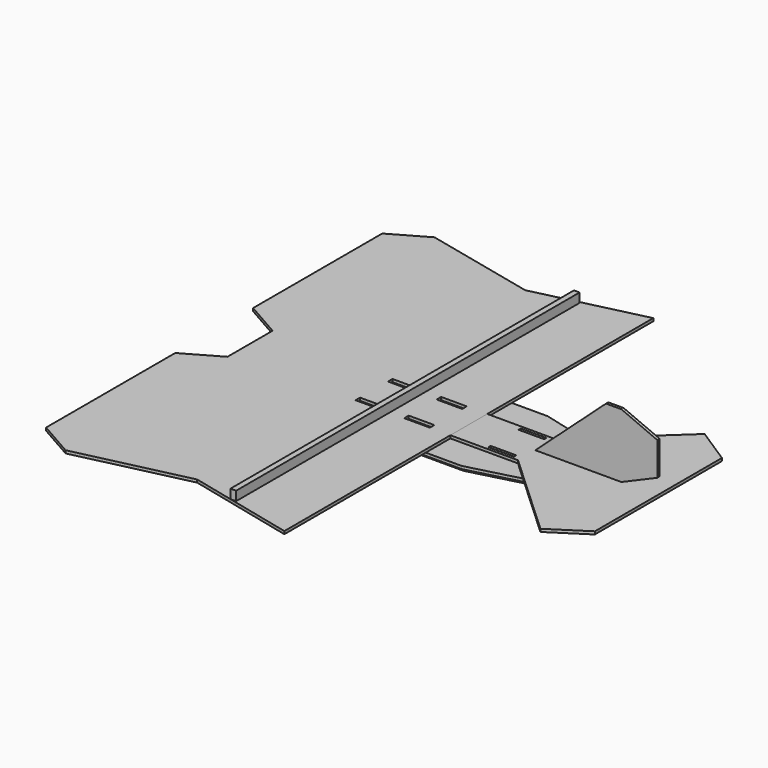
from build123d import *

# Parameters (mm, degrees)
F0_W      = 11
F0_H      = 50
F0_W_2    = 50
F0_H_2    = 11
F1_DEPTH  = 5.5
F2_W      = 11
F2_H      = 94.0476190476
F2_H_2    = 50
F2_H_3    = 110
F2_H_4    = 230
F3_DEPTH  = 18
F4_DEPTH  = 5.5
F5_W      = 50
F5_H      = 5.5
F5_W_2    = 120
F5_H_2    = 60
F6_DEPTH  = 5.5
F8_DEPTH  = 5.5
F9_W      = 50
F9_H      = 5.5
F9_W_2    = 40
F10_DEPTH = 5.5
F11_W     = 40
F11_H     = 5.5
F11_W_2   = 48
F11_W_3   = 20
F12_DEPTH = 125
F13_DEPTH = 5.5
F15_DEPTH = 5.5
F16_W     = 50
F16_H     = 5.5
F17_DEPTH = 5.5


# Not quite as in the source:
# - a feature names something its author has since deleted; it is built from what else it names


with BuildPart() as f1:
    # F0 (on Top) → F1 (new body)
    with BuildSketch(Plane.XY):
        Polygon((0, -400), (0, 0), (0, 400), (-217, 450), (-217, 400), (-217, 55), (-217, -55), (-217, -450), align=None)
        Polygon((-217, 400), (-217, 450), (-287, 410), (-287, 95), (-217, 55), align=None)
        Polygon((0, 400), (0, 0), (0, -400), (210, -450), (210, 0), (210, 450), align=None)
        with Locations((85.5, -300)):
            Rectangle(F0_W, F0_H, mode=Mode.SUBTRACT)
        with Locations((85.5, -140)):
            Rectangle(F0_W, F0_H, mode=Mode.SUBTRACT)
        with Locations((50, -39.5)):
            Rectangle(F0_W_2, F0_H_2, mode=Mode.SUBTRACT)
        with Locations((145, -39.5)):
            Rectangle(F0_W_2, F0_H_2, mode=Mode.SUBTRACT)
        with Locations((50, 39.5)):
            Rectangle(F0_W_2, F0_H_2, mode=Mode.SUBTRACT)
        with Locations((85.5, 140)):
            Rectangle(F0_W, F0_H, mode=Mode.SUBTRACT)
        with Locations((145, 39.5)):
            Rectangle(F0_W_2, F0_H_2, mode=Mode.SUBTRACT)
        with Locations((85.5, 300)):
            Rectangle(F0_W, F0_H, mode=Mode.SUBTRACT)
        Polygon((-287, -410), (-217, -450), (-217, -55), (-287, -95), align=None)
    extrude(amount=F1_DEPTH)


with BuildPart() as f3:
    # F2 (on face) → F3 (new body)
    with BuildSketch(Plane.XY.offset(5.5)):
        with Locations((85.5, -372.0238095238)):
            Rectangle(F2_W, F2_H)
        with Locations((85.5, -300)):
            Rectangle(F2_W, F2_H_2)
        with Locations((85.5, -220)):
            Rectangle(F2_W, F2_H_3)
        with Locations((85.5, -140)):
            Rectangle(F2_W, F2_H_2)
        with Locations((85.5, 0)):
            Rectangle(F2_W, F2_H_4)
        with Locations((85.5, 140)):
            Rectangle(F2_W, F2_H_2)
        with Locations((85.5, 220)):
            Rectangle(F2_W, F2_H_3)
        with Locations((85.5, 372.0238095238)):
            Rectangle(F2_W, F2_H)
        with Locations((85.5, 300)):
            Rectangle(F2_W, F2_H_2)
    extrude(amount=F3_DEPTH)

    # F0 (on Top) → F4 (join)
    with BuildSketch(Plane.XY):
        with Locations((85.5, -300)):
            Rectangle(F0_W, F0_H)
        with Locations((85.5, -140)):
            Rectangle(F0_W, F0_H)
        with Locations((85.5, 140)):
            Rectangle(F0_W, F0_H)
        with Locations((85.5, 300)):
            Rectangle(F0_W, F0_H)
    extrude(amount=F4_DEPTH)


with BuildPart() as f6:
    # F5 (on face) → F6 (new body)
    with BuildSketch(Plane.XY):
        Polygon((280, -105), (510, -45), (210, -45), (170, -45), (170, -34), (120, -34), (120, -45), (75, -45), (75, -34), (25, -34), (25, -45), (0, -45), (0, -105), align=None)
        Polygon((170, 34), (120, 34), (120, 45), (75, 45), (75, 34), (25, 34), (25, 45), (0, 45), (0, 0), (0, -45), (25, -45), (25, -34), (75, -34), (75, -45), (120, -45), (120, -34), (170, -34), (170, -45), (210, -45), (510, -45), (510, 0), (510, 45), (210, 45), (170, 45), align=None)
        with Locations((305, -36.75)):
            Rectangle(F5_W, F5_H, mode=Mode.SUBTRACT)
        with Locations((305, 36.75)):
            Rectangle(F5_W, F5_H, mode=Mode.SUBTRACT)
        Polygon((120, 45), (120, 34), (170, 34), (170, 45), (210, 45), (510, 45), (280, 105), (0, 105), (0, 45), (25, 45), (25, 34), (75, 34), (75, 45), align=None)
        with Locations((-60, 75)):
            Rectangle(F5_W_2, F5_H_2)
        Polygon((0, 0), (0, 45), (-120, 45), (-120, -45), (0, -45), align=None)
        with Locations((-60, -75)):
            Rectangle(F5_W_2, F5_H_2)
    extrude(amount=-F6_DEPTH)


with BuildPart() as f8:
    # F7 (on face) → F8 (new body)
    with BuildSketch(Plane(origin=(0, 0, -5.5), x_dir=(1, 0, 0), z_dir=(0, 0, -1))):
        Polygon((-120, 99.5), (-120, 50.5), (25, 50.5), (25, 39.5), (25, 34), (75, 34), (75, 39.5), (75, 50.5), (120, 50.5), (120, 39.5), (120, 34), (170, 34), (170, 39.5), (170, 50.5), (280, 50.5), (280, 39.5), (330, 39.5), (330, 50.5), (467.1277487393, 50.5), (279.294415406, 99.5), align=None)
    extrude(amount=F8_DEPTH)


with BuildPart() as f10:
    # F9 (on face) → F10 (new body)
    with BuildSketch(Plane.XY):
        Polygon((580, 155), (510, 200.2941176471), (510, 45), (510, 0), (510, -45), (510, -200.2941176471), (580, -155), (580, 0), align=None)
        Polygon((510, -45), (342, -45), (510, -200.2941176471), align=None)
        Polygon((342, 45), (210, 45), (210, -45), (342, -45), (510, -45), (510, 0), (510, 45), align=None)
        with Locations((305, -36.75)):
            Rectangle(F9_W, F9_H, mode=Mode.SUBTRACT)
        with Locations((382, 0)):
            Rectangle(F9_W_2, F9_H, mode=Mode.SUBTRACT)
        with Locations((470, 0)):
            Rectangle(F9_W_2, F9_H, mode=Mode.SUBTRACT)
        with Locations((305, 36.75)):
            Rectangle(F9_W, F9_H, mode=Mode.SUBTRACT)
        Polygon((510, 200.2941176471), (342, 45), (510, 45), align=None)
    extrude(amount=F10_DEPTH)


with BuildPart() as f12:
    # F11 (on face) → F12 (new body)
    with BuildSketch(Plane.XY.offset(5.5)):
        Polygon((490, 2.75), (490, -2.75), (510, -2.75), (510, 0), (510, 2.75), align=None)
        Polygon((510, 0), (510, -2.75), (580, -2.75), (580, 2.75), (510, 2.75), align=None)
        with Locations((470, 0)):
            Rectangle(F11_W, F11_H)
        with Locations((426, 0)):
            Rectangle(F11_W_2, F11_H)
        with Locations((382, 0)):
            Rectangle(F11_W, F11_H)
        with Locations((352, 0)):
            Rectangle(F11_W_3, F11_H)
    extrude(amount=F12_DEPTH)

    # F9 (on face) → F13 (join)
    with BuildSketch(Plane.XY):
        with Locations((470, 0)):
            Rectangle(F9_W_2, F9_H)
        with Locations((382, 0)):
            Rectangle(F9_W_2, F9_H)
    extrude(amount=F13_DEPTH)

    # F14 (on face) → F15 (cut, through all)
    with BuildSketch(Plane(origin=(0, 2.75, 0), x_dir=(-1, 0, 0), z_dir=(0, 1, 0))):
        Polygon((-580, 100.5), (-510, 130.5), (-580, 130.5), align=None)
        Polygon((-580, 5.5), (-510, 5.5), (-580, 35.5), align=None)
        Polygon((-342, 130.5), (-480, 130.5), (-342, 5.5), align=None)
    extrude(amount=-F15_DEPTH, mode=Mode.SUBTRACT)


with BuildPart() as f17:
    # F16 (on face) → F17 (new body)
    with BuildSketch(Plane(origin=(0, 0, -5.5), x_dir=(1, 0, 0), z_dir=(0, 0, -1))):
        Polygon((510, 39.5), (510, -39.5), (518, -39.5), (518, 0), (518, 39.5), align=None)
        with Locations((305, -36.75)):
            Rectangle(F16_W, F16_H)
        Polygon((330, -34), (330, -39.5), (510, -39.5), (510, 39.5), (330, 39.5), (330, 34), (280, 34), (280, -34), align=None)
        Polygon((-120, 0), (-120, -39.5), (280, -39.5), (280, -34), (280, 34), (280, 39.5), (-120, 39.5), align=None)
        with Locations((305, 36.75)):
            Rectangle(F16_W, F16_H)
    extrude(amount=F17_DEPTH)


solid = Compound([f1.part, f3.part, f6.part, f8.part, f10.part, f12.part, f17.part])
